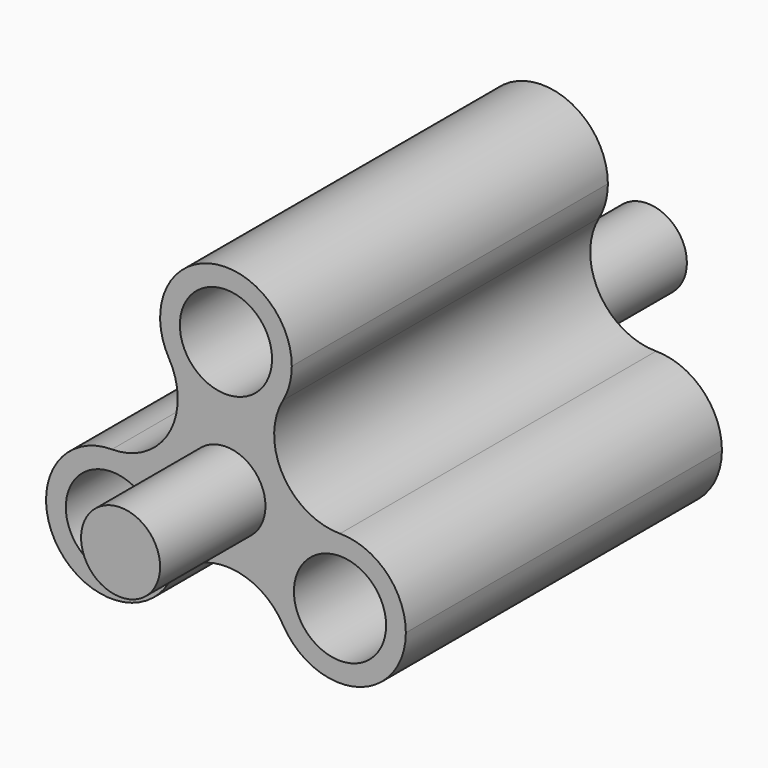
from build123d import *

# Parameters (mm, degrees)
F0_R          = 3.5
F1_DEPTH      = 30
F2_R          = 3
F3_DEPTH      = 40
F3_DEPTH_BACK = 10


# Not quite as in the source:
# - ends of sketch curves that miss each other by under 0.0002 mm in the source are joined


with BuildPart() as f1:
    # F0 (on Front) → F1 (new body)
    with BuildSketch(Plane.XZ):
        with BuildLine():
            ThreePointArc((-4.3301281481, 7.4999991798), (-6.557e-07, 5.0000002524), (4.330125744, 7.5000010726))
            ThreePointArc((4.330125744, 7.5000010726), (4.8296291409, 8.705905062), (5, 10.0000002524))
            ThreePointArc((5, 10.0000002524), (-1.2940954014, 14.8296293367), (-4.3301281481, 7.4999991798))
        make_face()
        with Locations((0, 10.0000002524)):
            Circle(F0_R, mode=Mode.SUBTRACT)
        with BuildLine():
            ThreePointArc((8.6602543293, 3.786e-07), (4.3301271646, 2.5000002524), (4.3301270553, 7.5000003155))
            ThreePointArc((4.3301270553, 7.5000003155), (-6.557e-07, 5.0000002524), (-4.3301281481, 7.4999991798))
            ThreePointArc((-4.3301281481, 7.4999991798), (-4.330127711, 2.499999306), (-8.6602543293, -1.1357e-06))
            ThreePointArc((-8.6602543293, -1.1357e-06), (-5.1247199995, -1.4644669979), (-3.6602536736, -5.0000011357))
            ThreePointArc((-3.6602536736, -5.0000011357), (-3.8306244761, -6.2940961149), (-4.3301263997, -7.500000694))
            ThreePointArc((-4.3301263997, -7.500000694), (4.371e-07, -5.0000002524), (4.330127711, -7.4999999369))
            ThreePointArc((4.330127711, -7.4999999369), (4.3301273832, -2.4999998738), (8.6602543293, 3.786e-07))
        make_face()
        with BuildLine():
            ThreePointArc((13.6602545478, -4.9999996214), (12.1957883765, -1.4644656382), (8.6602543293, 3.786e-07))
            ThreePointArc((8.6602543293, 3.786e-07), (4.3301273832, -2.4999998738), (4.330127711, -7.4999999369))
            ThreePointArc((4.330127711, -7.4999999369), (9.9543499492, -9.8296287058), (13.6602545478, -4.9999996214))
        make_face()
        with Locations((8.6602545478, -4.9999996214)):
            Circle(F0_R, mode=Mode.SUBTRACT)
        with BuildLine():
            ThreePointArc((-3.6602536736, -5.0000011357), (-5.1247199995, -1.4644669979), (-8.6602543293, -1.1357e-06))
            ThreePointArc((-8.6602543293, -1.1357e-06), (-12.9903804011, -7.5000016404), (-4.3301263997, -7.500000694))
            ThreePointArc((-4.3301263997, -7.500000694), (-3.8306244761, -6.2940961149), (-3.6602536736, -5.0000011357))
        make_face()
        with Locations((-8.6602536736, -5.0000011357)):
            Circle(F0_R, mode=Mode.SUBTRACT)
    extrude(amount=F1_DEPTH)

    # F2 (on Front) → F3 (join, two sides)
    with BuildSketch(Plane.XZ) as f3_sk:
        Circle(F2_R)
    extrude(amount=F3_DEPTH)
    extrude(f3_sk.sketch, amount=-F3_DEPTH_BACK)


solid = f1.part
